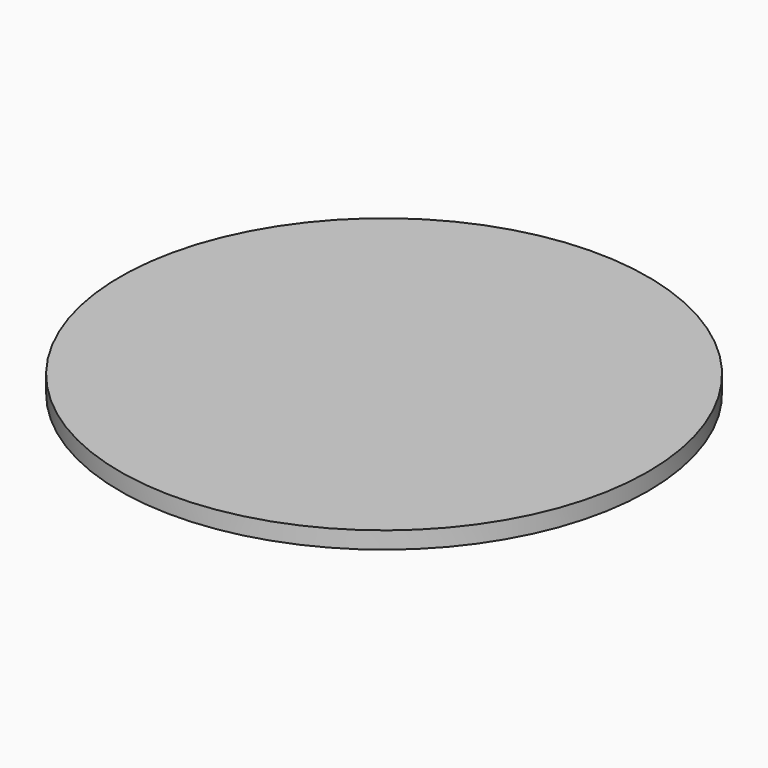
from build123d import *

# Parameters (mm, degrees)
F0_R     = 31
F1_DEPTH = 2


# Not quite as in the source:
# - the program builds the solid bodies; features that only make, move or delete a surface that nothing else refers to are left out


with BuildPart() as f1:
    # F0 (on Top) → F1 (new body)
    with BuildSketch(Plane.XY):
        Circle(F0_R)
    extrude(amount=F1_DEPTH)


solid = f1.part
